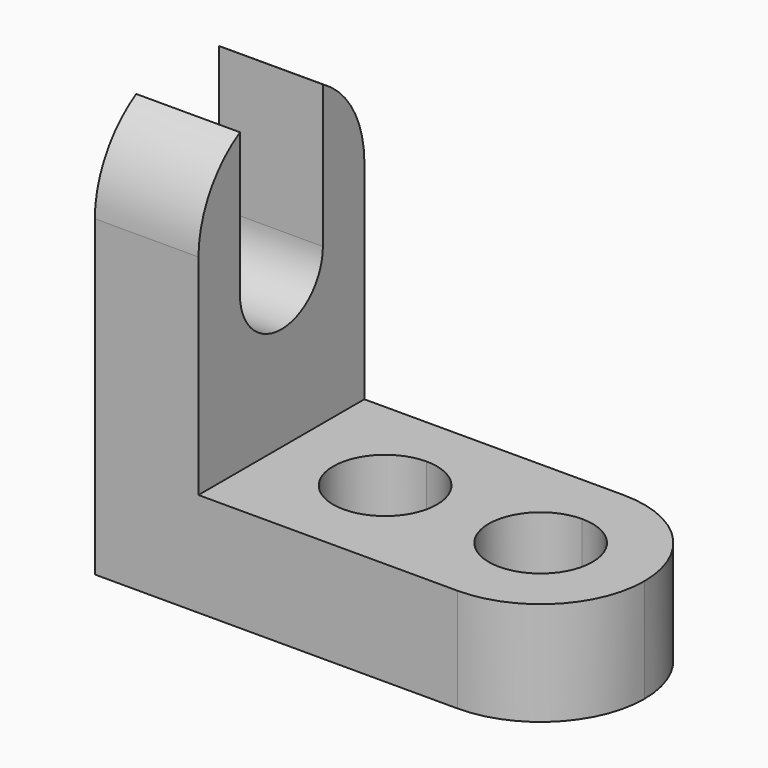
from build123d import *

# Parameters (mm, degrees)
F1_DEPTH = 25.4
F3_DEPTH = 12.701
F5_DEPTH = 12.701
F7_DEPTH = 12.701


with BuildPart() as f1:
    # F0 (on Front) → F1 (new body)
    with BuildSketch(Plane.XZ):
        Polygon((0, 50.8), (0, 0), (57.15, 0), (57.15, 12.7), (12.7, 12.7), (12.7, 50.8), align=None)
    extrude(amount=F1_DEPTH)

    # F2 (on face) → F3 (cut, through all)
    with BuildSketch(Plane.YZ.offset(12.7)):
        with BuildLine():
            ThreePointArc((-6.35, 31.75), (-12.7, 38.1), (-19.05, 31.75))
            Line((-19.05, 31.75), (-6.35, 31.75))
        make_face()
        with BuildLine():
            Line((-6.35, 31.75), (-19.05, 31.75))
            ThreePointArc((-19.05, 31.75), (-12.7, 25.4), (-6.35, 31.75))
        make_face()
        with BuildLine():
            Line((-19.05, 50.8), (-19.05, 31.75))
            ThreePointArc((-19.05, 31.75), (-12.7, 38.1), (-6.35, 31.75))
            Line((-6.35, 31.75), (-6.35, 50.8))
            Line((-6.35, 50.8), (-19.05, 50.8))
        make_face()
    extrude(amount=-F3_DEPTH, mode=Mode.SUBTRACT)

    # F4 (on face) → F5 (cut, through all)
    with BuildSketch(Plane.YZ.offset(12.7)):
        with BuildLine():
            Line((-25.4, 50.8), (-25.4, 38.3654093824))
            ThreePointArc((-25.4, 38.3654093824), (-23.6656953438, 44.6406010825), (-19.05, 49.2320278765))
            Line((-19.05, 49.2320278765), (-19.05, 50.8))
            Line((-19.05, 50.8), (-25.4, 50.8))
        make_face()
        with BuildLine():
            Line((-6.35, 50.8), (-6.35, 49.2320278765))
            ThreePointArc((-6.35, 49.2320278765), (-1.7343046562, 44.6406010825), (0, 38.3654093824))
            Line((0, 38.3654093824), (0, 50.8))
            Line((0, 50.8), (-6.35, 50.8))
        make_face()
    extrude(amount=-F5_DEPTH, mode=Mode.SUBTRACT)

    # F6 (on face) → F7 (cut, through all)
    with BuildSketch(Plane.XY.offset(12.7)):
        with BuildLine():
            ThreePointArc((25.4, -6.35), (19.05, -12.7), (25.4, -19.05))
            Line((25.4, -19.05), (25.4, -6.35))
        make_face()
        with BuildLine():
            Line((25.4, -6.35), (25.4, -19.05))
            ThreePointArc((25.4, -19.05), (29.8901280605, -17.1901280605), (31.75, -12.7))
            ThreePointArc((31.75, -12.7), (29.8901280605, -8.2098719395), (25.4, -6.35))
        make_face()
        with BuildLine():
            ThreePointArc((44.45, -6.35), (38.1, -12.7), (44.45, -19.05))
            Line((44.45, -19.05), (44.45, -6.35))
        make_face()
        with BuildLine():
            Line((44.45, -6.35), (44.45, -19.05))
            ThreePointArc((44.45, -19.05), (48.9401280605, -17.1901280605), (50.8, -12.7))
            ThreePointArc((50.8, -12.7), (48.9401280605, -8.2098719395), (44.45, -6.35))
        make_face()
        with BuildLine():
            ThreePointArc((57.15, -12.7), (53.4302561211, -21.6802561211), (44.45, -25.4))
            Line((44.45, -25.4), (57.15, -25.4))
            Line((57.15, -25.4), (57.15, -12.7))
        make_face()
        with BuildLine():
            ThreePointArc((44.45, 0), (53.4302561211, -3.7197438789), (57.15, -12.7))
            Line((57.15, -12.7), (57.15, 0))
            Line((57.15, 0), (44.45, 0))
        make_face()
    extrude(amount=-F7_DEPTH, mode=Mode.SUBTRACT)


solid = f1.part
